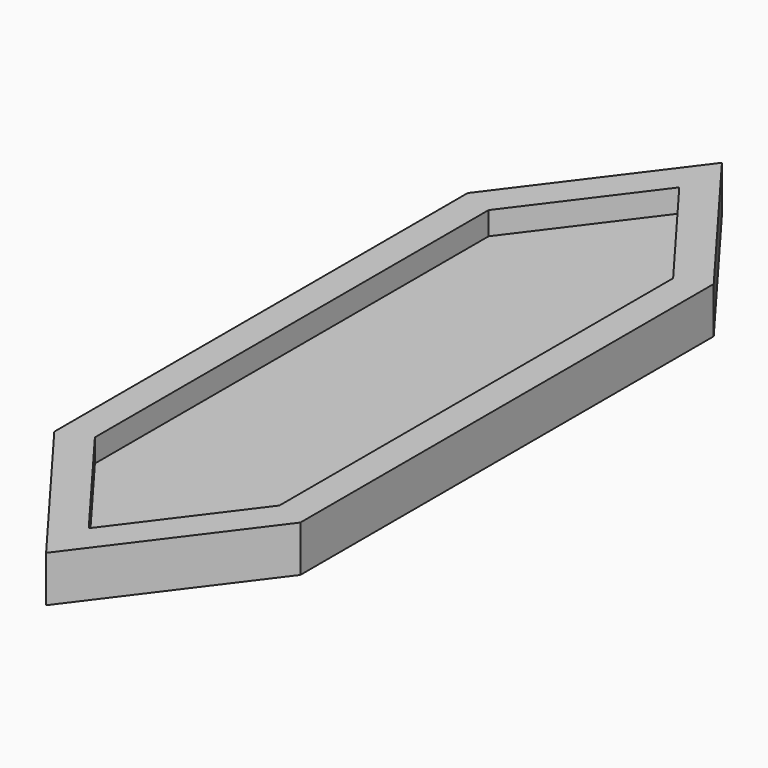
from build123d import *

# Parameters (mm, degrees)
F1_DEPTH = 9.525
F2_DEPTH = 4.7625


# Not quite as in the source:
# - a feature names something its author has since deleted; it is built from what else it names


with BuildPart() as f1:
    # F0 (on Top) → F1 (new body)
    with BuildSketch(Plane.XY):
        Polygon((0, 87.2066666667), (-25.4, 53.34), (-25.4, -53.34), (0, -87.2066666667), (25.4, -53.34), (25.4, 53.34), align=None)
        Polygon((-19.05, -50.8), (-19.05, 50.8), (0, 76.2), (19.05, 50.8), (19.05, -50.8), (0, -76.2), align=None, mode=Mode.SUBTRACT)
    extrude(amount=F1_DEPTH)

    # F0 (on Top) → F2 (join)
    with BuildSketch(Plane.XY):
        Polygon((0, 76.2), (-19.05, 50.8), (-19.05, -50.8), (0, -76.2), (19.05, -50.8), (19.05, 50.8), align=None)
    extrude(amount=F2_DEPTH)


solid = f1.part
